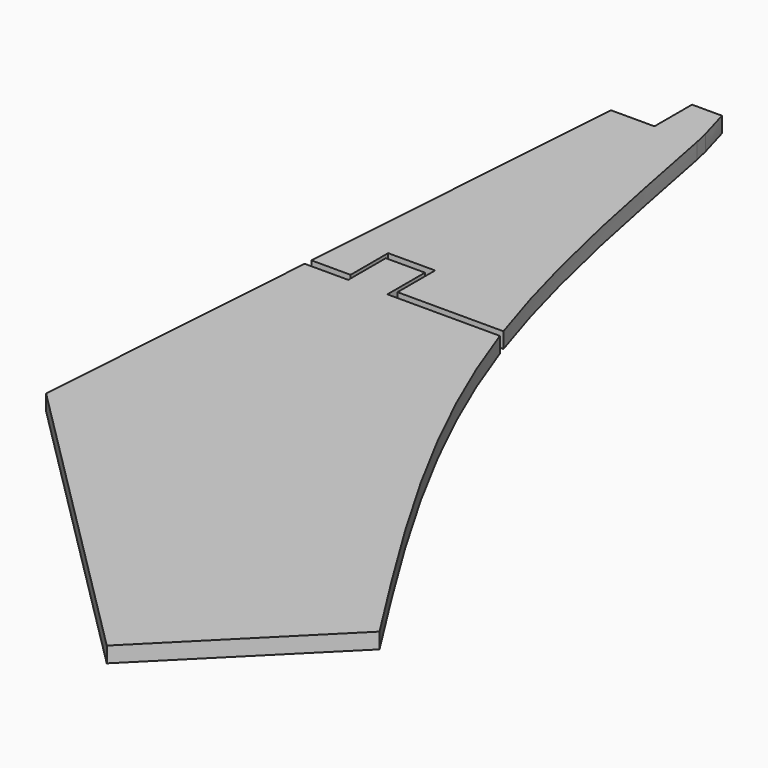
from build123d import *

# Parameters (mm, degrees)
F1_DEPTH = 2


with BuildPart() as f1:
    # F0 (on Top) → F1 (new body)
    with BuildSketch(Plane.XY):
        with BuildLine():
            Line((-36.1030085053, -18.1074753944), (-38.7452475978, -56.1074753944))
            Line((-38.7452475978, -56.1074753944), (0.0209415142, -94.8736645064))
            Line((0.0209415142, -94.8736645064), (19.383590258, -75.5110157627))
            add(Edge.make_bspline(
                [(-11.1606838182, -18.1079245215), (-3.9272930935, -38.8901161994), (7.7283923455, -57.2005538635), (19.383590258, -75.5110157627)],
                knots=[0.5354752701, 0.5354752701, 0.5354752701, 0.5354752701, 1, 1, 1, 1], degree=3))
            Line((-11.1606838182, -18.1079245215), (-25.5334842512, -18.1079245215))
            Line((-25.5334842512, -18.1079245215), (-25.5334842512, -12.1074753944))
            Line((-25.5334842512, -12.1074753944), (-30.5334842512, -12.1074753944))
            Line((-30.5334842512, -12.1074753944), (-30.5334842512, -18.1074753944))
            Line((-30.5334842512, -18.1074753944), (-36.1030085053, -18.1074753944))
        make_face()
    extrude(amount=F1_DEPTH)


with BuildPart() as f1b:
    # F0 (on Top) → F1, piece 2 (new body)
    with BuildSketch(Plane.XY):
        with BuildLine():
            Line((-25.0334758969, -17.1079245215), (-11.5047290727, -17.1079056856))
            add(Edge.make_bspline(
                [(-21.9740723878, 26.8920754785), (-20.2514084677, 18.872572648), (-17.3749052233, 0.1533534673), (-11.5047290727, -17.1079056856)],
                knots=[0.1435758268, 0.1435758268, 0.1435758268, 0.1435758268, 0.5280379508, 0.5280379508, 0.5280379508, 0.5280379508], degree=3))
            Line((-21.9740723878, 26.8920754785), (-22.404534184, 26.8920754785))
            Line((-22.404534184, 26.8920754785), (-27.404534184, 26.8920754785))
            Line((-27.404534184, 26.8920754785), (-32.9740723878, 26.8920754785))
            Line((-32.9740723878, 26.8920754785), (-36.0334758976, -17.1074753944))
            Line((-36.0334758976, -17.1074753944), (-31.0334758976, -17.1074753944))
            Line((-31.0334758976, -17.1074753944), (-31.0334842512, -11.1074753944))
            Line((-31.0334842512, -11.1074753944), (-25.0334842513, -11.1074670407))
            Line((-25.0334842513, -11.1074670407), (-25.0334758969, -17.1079245215))
        make_face()
        with BuildLine():
            Line((-22.404534184, 26.8920754785), (-21.9740723878, 26.8920754785))
            add(Edge.make_bspline(
                [(-22.404534184, 28.7817309061), (-22.2685909811, 28.2218066684), (-22.1258076558, 27.598447393), (-21.9740723878, 26.8920754785)],
                knots=[0.1097117267, 0.1097117267, 0.1097117267, 0.1097117267, 0.1435758268, 0.1435758268, 0.1435758268, 0.1435758268], degree=3))
            Line((-22.404534184, 28.7817309061), (-22.404534184, 26.8920754785))
        make_face()
        with BuildLine():
            Line((-27.404534184, 26.8920754785), (-22.404534184, 26.8920754785))
            Line((-22.404534184, 26.8920754785), (-22.404534184, 28.7817309061))
            add(Edge.make_bspline(
                [(-23.5822349949, 32.8920754785), (-23.213587795, 31.7439577547), (-22.8449582167, 30.5957538617), (-22.404534184, 28.7817309061)],
                knots=[0, 0, 0, 0, 0.1097117267, 0.1097117267, 0.1097117267, 0.1097117267], degree=3))
            Line((-23.5822349949, 32.8920754785), (-27.404534184, 32.8920754785))
            Line((-27.404534184, 32.8920754785), (-27.404534184, 26.8920754785))
        make_face()
    extrude(amount=F1_DEPTH)


solid = Compound([f1.part, f1b.part])
